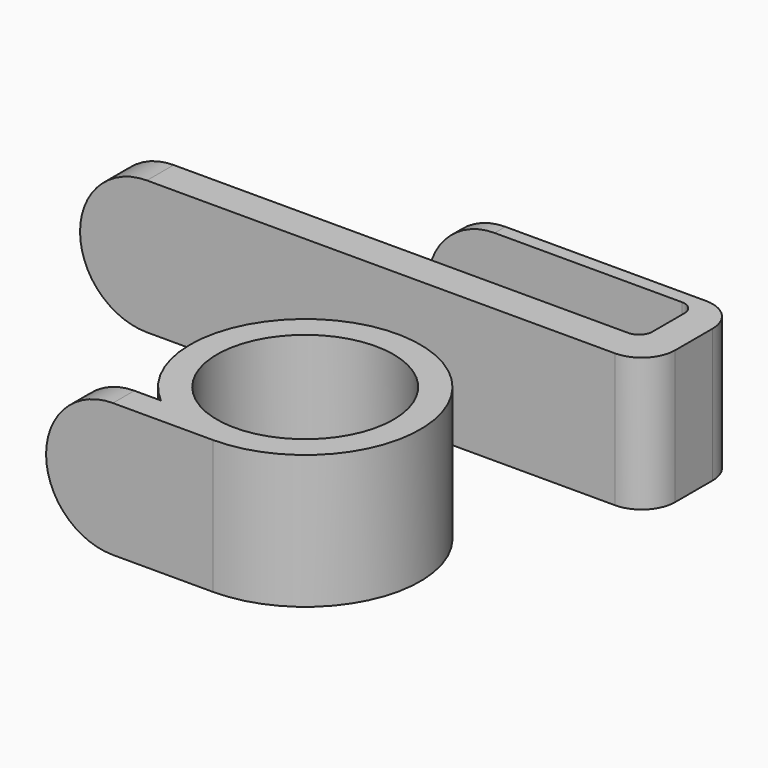
from build123d import *

# Parameters (mm, degrees)
F0_R     = 21.844
F0_R_2   = 16.764
F1_DEPTH = 25.4
F3_W     = 19.05
F3_H     = 25.4
F4_DEPTH = 5.08
F6_DEPTH = 25.4
F7_R     = 12.69999


# Not quite as in the source:
# - a fillet or chamfer is up to 0.001 mm smaller than in the source, because OpenCascade refuses the exact size


with BuildPart() as f1:
    # F0 (on Top) → F1 (new body)
    with BuildSketch(Plane.XY):
        Circle(F0_R)
        Circle(F0_R_2, mode=Mode.SUBTRACT)
    extrude(amount=F1_DEPTH)

    # F3 (on offset) → F4 (join)
    with BuildSketch(Plane.XZ.offset(21.844)):
        with Locations((-9.525, 12.7)):
            Rectangle(F3_W, F3_H)
        with BuildLine():
            ThreePointArc((-19.05, 25.4), (-31.75, 12.7), (-19.05, 0))
            Line((-19.05, 0), (-19.05, 25.4))
        make_face()
    extrude(amount=-F4_DEPTH)


with BuildPart() as f6:
    # F5 (on Top) → F6 (new body)
    with BuildSketch(Plane.XY):
        with BuildLine():
            ThreePointArc((29.1176303876, 46.0293454591), (28.3736816118, 44.2332942349), (26.5776303876, 43.4893454591))
            Line((26.5776303876, 43.4893454591), (-72.4823696124, 43.4893454591))
            Line((-72.4823696124, 43.4893454591), (-72.4823696124, 37.1393454591))
            Line((-72.4823696124, 37.1393454591), (29.1176303876, 37.1393454591))
            ThreePointArc((29.1176303876, 37.1393454591), (33.6077584481, 38.9992173986), (35.4676303876, 43.4893454591))
            Line((35.4676303876, 43.4893454591), (35.4676303876, 52.3793454591))
            ThreePointArc((35.4676303876, 52.3793454591), (33.6077584481, 56.8694735197), (29.1176303876, 58.7293454591))
            Line((29.1176303876, 58.7293454591), (-21.6823696124, 58.7293454591))
            Line((-21.6823696124, 58.7293454591), (-21.6823696124, 56.1893454591))
            Line((-21.6823696124, 56.1893454591), (26.5776303876, 56.1893454591))
            ThreePointArc((26.5776303876, 56.1893454591), (28.3736816118, 55.4453966833), (29.1176303876, 53.6493454591))
            Line((29.1176303876, 53.6493454591), (29.1176303876, 46.0293454591))
        make_face()
    extrude(amount=F6_DEPTH)

    # F7 (radius 12.7 in the source; OpenCascade refuses exactly that, so slightly less here)
    f7_edges = [f6.edges().sort_by_distance(p)[0] for p in [
        (-72.48237, 40.314345, 25.4),
        (-72.48237, 40.314345, 0),
        (-21.68237, 57.459345, 25.4),
        (-21.68237, 57.459345, 0),
    ]]
    fillet(f7_edges, radius=F7_R)


solid = Compound([f1.part, f6.part])
